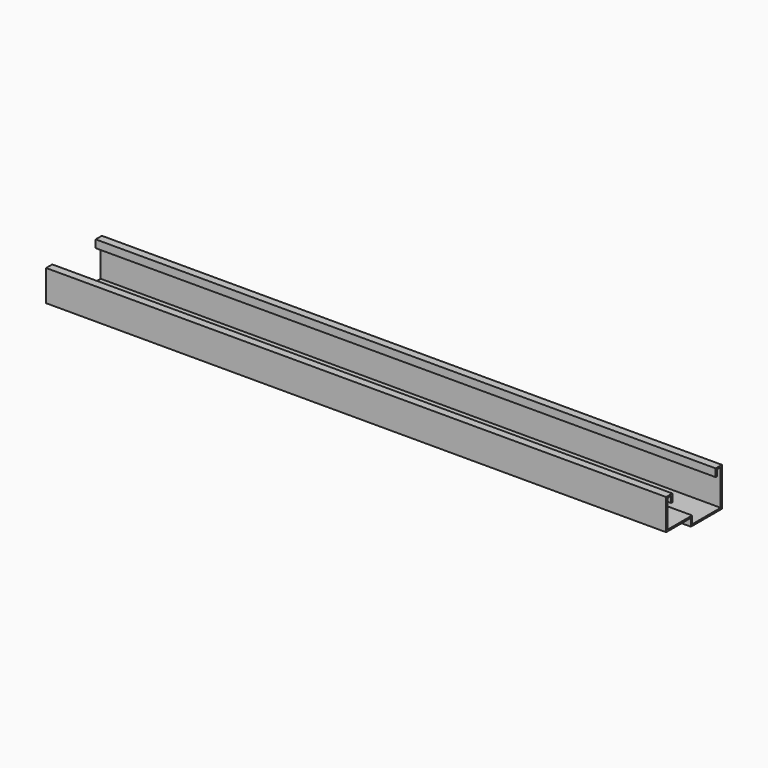
from build123d import *

# Parameters (mm, degrees)
F1_DEPTH = 800
F2_ANGLE = 180
F3_ANGLE = 270


# Not quite as in the source:
# - a feature of the source that left no trace in its solid (it failed there, or was rolled back) is left out


with BuildPart() as f1:
    # F0 (on Top) → F1 (new body)
    with BuildSketch(Plane.XY):
        Polygon((10, 0), (0, 0), (0, -10), (40, -10), (40, 30), (50, 30), (50, 80), (0, 80), (0, 70), (10, 70), (10, 72), (2.000000095, 72), (2.000000095, 78), (48, 78), (48, 32), (38, 32), (38, -8), (2, -8), (2, -2), (10, -2), align=None)
    extrude(amount=F1_DEPTH)


with BuildPart() as f1_1:
    # F2: moved
    add(f1.part.rotate(Axis((50, 55, 800), (0, 1, 0)), F2_ANGLE))


with BuildPart() as f1_2:
    # F3: moved
    add(f1_1.part.rotate(Axis((50, 55, 800), (0, 1, 0)), F3_ANGLE))


solid = f1_2.part
